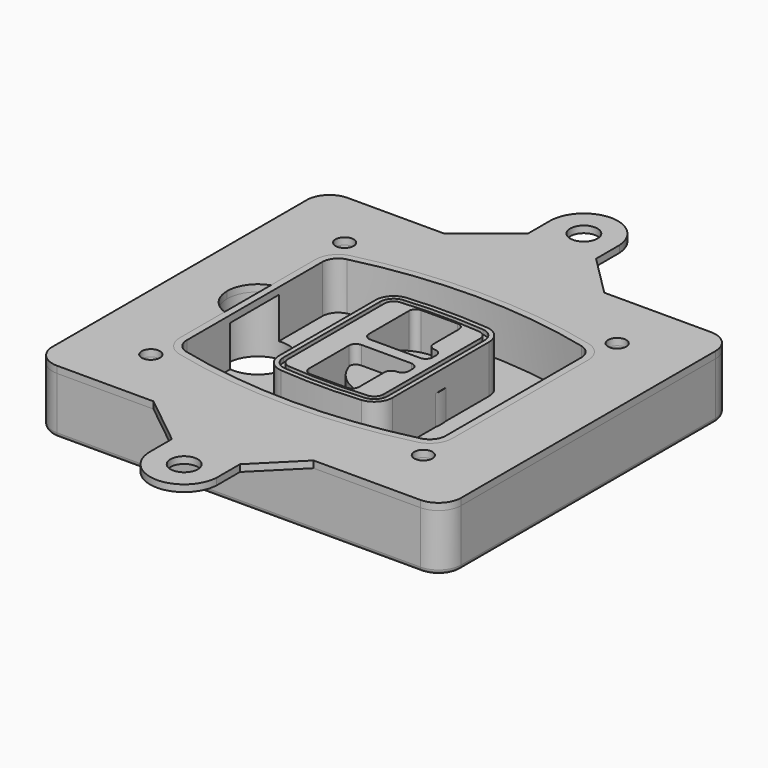
from build123d import *

# Parameters (mm, degrees)
F0_R      = 4
F1_DEPTH  = 25
F2_DEPTH  = 3
F3_DEPTH  = 18
F5_DEPTH  = 21
F6_DEPTH  = 2
F8_DEPTH  = 20
F9_DEPTH  = 16
F10_DEPTH = 25
F7_R      = 6
F7_R_2    = 4
F11_DEPTH = 6
F13_DEPTH = 9
F15_R     = 2
F16_R     = 6
F16_R_2   = 4
F17_DEPTH = 3


# Not quite as in the source:
# - a feature of the source that left no trace in its solid (it failed there, or was rolled back) is left out
# - a feature names something its author has since deleted; it is built from what else it names


with BuildPart() as f1:
    # F0 (on Top) → F1 (new body)
    with BuildSketch(Plane.XY):
        with BuildLine():
            ThreePointArc((-90, -70), (-87.0710678119, -77.0710678119), (-80, -80))
            Line((-80, -80), (80, -80))
            ThreePointArc((80, -80), (87.0710678119, -77.0710678119), (90, -70))
            Line((90, -70), (90, 70))
            ThreePointArc((90, 70), (87.0710678119, 77.0710678119), (80, 80))
            Line((80, 80), (-80, 80))
            ThreePointArc((-80, 80), (-87.0710678119, 77.0710678119), (-90, 70))
            Line((-90, 70), (-90, -70))
        make_face()
        with Locations((-60, -53.3333333333)):
            Circle(F0_R, mode=Mode.SUBTRACT)
        with Locations((60, -53.3333333333)):
            Circle(F0_R, mode=Mode.SUBTRACT)
        with Locations((-60, 53.3333333333)):
            Circle(F0_R, mode=Mode.SUBTRACT)
        with BuildLine():
            ThreePointArc((-64, 37.2990447398), (-61.0143011354, 45.9411029726), (-53.3306899286, 50.8970778549))
            ThreePointArc((-53.3306899286, 50.8970778549), (0, 57.3333333333), (53.3306899286, 50.8970778549))
            ThreePointArc((53.3306899286, 50.8970778549), (61.0143011354, 45.9411029726), (64, 37.2990447398))
            Line((64, 37.2990447398), (64, -37.2990447398))
            ThreePointArc((64, -37.2990447398), (61.0143011354, -45.9411029726), (53.3306899286, -50.8970778549))
            ThreePointArc((53.3306899286, -50.8970778549), (0, -57.3333333333), (-53.3306899286, -50.8970778549))
            ThreePointArc((-53.3306899286, -50.8970778549), (-61.0143011354, -45.9411029726), (-64, -37.2990447398))
            Line((-64, -37.2990447398), (-64, 37.2990447398))
        make_face(mode=Mode.SUBTRACT)
        with Locations((60, 53.3333333333)):
            Circle(F0_R, mode=Mode.SUBTRACT)
        with BuildLine():
            ThreePointArc((53.3306899286, 50.8970778549), (0, 57.3333333333), (-53.3306899286, 50.8970778549))
            ThreePointArc((-53.3306899286, 50.8970778549), (-61.0143011354, 45.9411029726), (-64, 37.2990447398))
            Line((-64, 37.2990447398), (-64, -37.2990447398))
            ThreePointArc((-64, -37.2990447398), (-61.0143011354, -45.9411029726), (-53.3306899286, -50.8970778549))
            ThreePointArc((-53.3306899286, -50.8970778549), (0, -57.3333333333), (53.3306899286, -50.8970778549))
            ThreePointArc((53.3306899286, -50.8970778549), (61.0143011354, -45.9411029726), (64, -37.2990447398))
            Line((64, -37.2990447398), (64, 37.2990447398))
            ThreePointArc((64, 37.2990447398), (61.0143011354, 45.9411029726), (53.3306899286, 50.8970778549))
        make_face()
        with BuildLine():
            Line((-60, -37.2990447398), (-60, 37.2990447398))
            ThreePointArc((-60, 37.2990447398), (-57.8673579538, 43.4719434775), (-52.3790642347, 47.0119255363))
            ThreePointArc((-52.3790642347, 47.0119255363), (0, 53.3333333333), (52.3790642347, 47.0119255363))
            ThreePointArc((52.3790642347, 47.0119255363), (57.8673579538, 43.4719434775), (60, 37.2990447398))
            Line((60, 37.2990447398), (60, -37.2990447398))
            ThreePointArc((60, -37.2990447398), (57.8673579538, -43.4719434775), (52.3790642347, -47.0119255363))
            ThreePointArc((52.3790642347, -47.0119255363), (0, -53.3333333333), (-52.3790642347, -47.0119255363))
            ThreePointArc((-52.3790642347, -47.0119255363), (-57.8673579538, -43.4719434775), (-60, -37.2990447398))
        make_face(mode=Mode.SUBTRACT)
        with BuildLine():
            ThreePointArc((-52.3790642347, 47.0119255363), (-57.8673579538, 43.4719434775), (-60, 37.2990447398))
            Line((-60, 37.2990447398), (-60, -37.2990447398))
            ThreePointArc((-60, -37.2990447398), (-57.8673579538, -43.4719434775), (-52.3790642347, -47.0119255363))
            ThreePointArc((-52.3790642347, -47.0119255363), (0, -53.3333333333), (52.3790642347, -47.0119255363))
            ThreePointArc((52.3790642347, -47.0119255363), (57.8673579538, -43.4719434775), (60, -37.2990447398))
            Line((60, -37.2990447398), (60, 37.2990447398))
            ThreePointArc((60, 37.2990447398), (57.8673579538, 43.4719434775), (52.3790642347, 47.0119255363))
            ThreePointArc((52.3790642347, 47.0119255363), (0, 53.3333333333), (-52.3790642347, 47.0119255363))
        make_face()
        with BuildLine():
            ThreePointArc((51.6653449643, 44.0980612973), (55.5071505677, 41.6200738562), (57, 37.2990447398))
            Line((57, 37.2990447398), (57, -37.2990447398))
            ThreePointArc((57, -37.2990447398), (55.5071505677, -41.6200738562), (51.6653449643, -44.0980612973))
            ThreePointArc((51.6653449643, -44.0980612973), (0, -50.3333333333), (-51.6653449643, -44.0980612973))
            ThreePointArc((-51.6653449643, -44.0980612973), (-55.5071505677, -41.6200738562), (-57, -37.2990447398))
            Line((-57, -37.2990447398), (-57, 37.2990447398))
            ThreePointArc((-57, 37.2990447398), (-55.5071505677, 41.6200738562), (-51.6653449643, 44.0980612973))
            ThreePointArc((-51.6653449643, 44.0980612973), (0, 50.3333333333), (51.6653449643, 44.0980612973))
        make_face(mode=Mode.SUBTRACT)
        with BuildLine():
            Line((57, -37.2990447398), (57, 37.2990447398))
            ThreePointArc((57, 37.2990447398), (55.5071505677, 41.6200738562), (51.6653449643, 44.0980612973))
            ThreePointArc((51.6653449643, 44.0980612973), (0, 50.3333333333), (-51.6653449643, 44.0980612973))
            ThreePointArc((-51.6653449643, 44.0980612973), (-55.5071505677, 41.6200738562), (-57, 37.2990447398))
            Line((-57, 37.2990447398), (-57, -37.2990447398))
            ThreePointArc((-57, -37.2990447398), (-55.5071505677, -41.6200738562), (-51.6653449643, -44.0980612973))
            ThreePointArc((-51.6653449643, -44.0980612973), (0, -50.3333333333), (51.6653449643, -44.0980612973))
            ThreePointArc((51.6653449643, -44.0980612973), (55.5071505677, -41.6200738562), (57, -37.2990447398))
        make_face()
    extrude(amount=-F1_DEPTH)

    # F0 (on Top) → F2 (join)
    with BuildSketch(Plane.XY):
        with BuildLine():
            ThreePointArc((-52.3790642347, 47.0119255363), (-57.8673579538, 43.4719434775), (-60, 37.2990447398))
            Line((-60, 37.2990447398), (-60, -37.2990447398))
            ThreePointArc((-60, -37.2990447398), (-57.8673579538, -43.4719434775), (-52.3790642347, -47.0119255363))
            ThreePointArc((-52.3790642347, -47.0119255363), (0, -53.3333333333), (52.3790642347, -47.0119255363))
            ThreePointArc((52.3790642347, -47.0119255363), (57.8673579538, -43.4719434775), (60, -37.2990447398))
            Line((60, -37.2990447398), (60, 37.2990447398))
            ThreePointArc((60, 37.2990447398), (57.8673579538, 43.4719434775), (52.3790642347, 47.0119255363))
            ThreePointArc((52.3790642347, 47.0119255363), (0, 53.3333333333), (-52.3790642347, 47.0119255363))
        make_face()
        with BuildLine():
            ThreePointArc((51.6653449643, 44.0980612973), (55.5071505677, 41.6200738562), (57, 37.2990447398))
            Line((57, 37.2990447398), (57, -37.2990447398))
            ThreePointArc((57, -37.2990447398), (55.5071505677, -41.6200738562), (51.6653449643, -44.0980612973))
            ThreePointArc((51.6653449643, -44.0980612973), (0, -50.3333333333), (-51.6653449643, -44.0980612973))
            ThreePointArc((-51.6653449643, -44.0980612973), (-55.5071505677, -41.6200738562), (-57, -37.2990447398))
            Line((-57, -37.2990447398), (-57, 37.2990447398))
            ThreePointArc((-57, 37.2990447398), (-55.5071505677, 41.6200738562), (-51.6653449643, 44.0980612973))
            ThreePointArc((-51.6653449643, 44.0980612973), (0, 50.3333333333), (51.6653449643, 44.0980612973))
        make_face(mode=Mode.SUBTRACT)
    extrude(amount=F2_DEPTH)

    # F0 (on Top) → F3 (cut)
    with BuildSketch(Plane.XY):
        with BuildLine():
            Line((57, -37.2990447398), (57, 37.2990447398))
            ThreePointArc((57, 37.2990447398), (55.5071505677, 41.6200738562), (51.6653449643, 44.0980612973))
            ThreePointArc((51.6653449643, 44.0980612973), (0, 50.3333333333), (-51.6653449643, 44.0980612973))
            ThreePointArc((-51.6653449643, 44.0980612973), (-55.5071505677, 41.6200738562), (-57, 37.2990447398))
            Line((-57, 37.2990447398), (-57, -37.2990447398))
            ThreePointArc((-57, -37.2990447398), (-55.5071505677, -41.6200738562), (-51.6653449643, -44.0980612973))
            ThreePointArc((-51.6653449643, -44.0980612973), (0, -50.3333333333), (51.6653449643, -44.0980612973))
            ThreePointArc((51.6653449643, -44.0980612973), (55.5071505677, -41.6200738562), (57, -37.2990447398))
        make_face()
    extrude(amount=-F3_DEPTH, mode=Mode.SUBTRACT)

    # F4 (on face) → F5 (join, through all)
    with BuildSketch(Plane.XY.offset(3)):
        with BuildLine():
            ThreePointArc((-25, -26.587695628), (-22.8992979869, -31.9912392117), (-17.7004291845, -34.5569740744))
            ThreePointArc((-17.7004291845, -34.5569740744), (0, -35.3333333333), (17.7004291845, -34.5569740744))
            ThreePointArc((17.7004291845, -34.5569740744), (22.8992979869, -31.9912392117), (25, -26.587695628))
            Line((25, -26.587695628), (25, 26.587695628))
            ThreePointArc((25, 26.587695628), (22.8992979869, 31.9912392117), (17.7004291845, 34.5569740744))
            ThreePointArc((17.7004291845, 34.5569740744), (0, 35.3333333333), (-17.7004291845, 34.5569740744))
            ThreePointArc((-17.7004291845, 34.5569740744), (-22.8992979869, 31.9912392117), (-25, 26.587695628))
            Line((-25, 26.587695628), (-25, -26.587695628))
        make_face()
        with BuildLine():
            ThreePointArc((17.5253218884, 32.5646544628), (21.4244734902, 30.6403533158), (23, 26.587695628))
            Line((23, 26.587695628), (23, -26.587695628))
            ThreePointArc((23, -26.587695628), (21.4244734902, -30.6403533158), (17.5253218884, -32.5646544628))
            ThreePointArc((17.5253218884, -32.5646544628), (0, -33.3333333333), (-17.5253218884, -32.5646544628))
            ThreePointArc((-17.5253218884, -32.5646544628), (-21.4244734902, -30.6403533158), (-23, -26.587695628))
            Line((-23, -26.587695628), (-23, 26.587695628))
            ThreePointArc((-23, 26.587695628), (-21.4244734902, 30.6403533158), (-17.5253218884, 32.5646544628))
            ThreePointArc((-17.5253218884, 32.5646544628), (0, 33.3333333333), (17.5253218884, 32.5646544628))
        make_face(mode=Mode.SUBTRACT)
        with BuildLine():
            Line((23, -26.587695628), (23, 26.587695628))
            ThreePointArc((23, 26.587695628), (21.4244734902, 30.6403533158), (17.5253218884, 32.5646544628))
            ThreePointArc((17.5253218884, 32.5646544628), (0, 33.3333333333), (-17.5253218884, 32.5646544628))
            ThreePointArc((-17.5253218884, 32.5646544628), (-21.4244734902, 30.6403533158), (-23, 26.587695628))
            Line((-23, 26.587695628), (-23, -26.587695628))
            ThreePointArc((-23, -26.587695628), (-21.4244734902, -30.6403533158), (-17.5253218884, -32.5646544628))
            ThreePointArc((-17.5253218884, -32.5646544628), (0, -33.3333333333), (17.5253218884, -32.5646544628))
            ThreePointArc((17.5253218884, -32.5646544628), (21.4244734902, -30.6403533158), (23, -26.587695628))
        make_face()
        with BuildLine():
            ThreePointArc((17.3502145923, 30.5723348512), (19.9496489934, 29.2894674198), (21, 26.587695628))
            Line((21, 26.587695628), (21, -26.587695628))
            ThreePointArc((21, -26.587695628), (19.9496489934, -29.2894674198), (17.3502145923, -30.5723348512))
            ThreePointArc((17.3502145923, -30.5723348512), (0, -31.3333333333), (-17.3502145923, -30.5723348512))
            ThreePointArc((-17.3502145923, -30.5723348512), (-19.9496489934, -29.2894674198), (-21, -26.587695628))
            Line((-21, -26.587695628), (-21, 26.587695628))
            ThreePointArc((-21, 26.587695628), (-19.9496489934, 29.2894674198), (-17.3502145923, 30.5723348512))
            ThreePointArc((-17.3502145923, 30.5723348512), (0, 31.3333333333), (17.3502145923, 30.5723348512))
        make_face(mode=Mode.SUBTRACT)
        with BuildLine():
            Line((21, -26.587695628), (21, 26.587695628))
            ThreePointArc((21, 26.587695628), (19.9496489934, 29.2894674198), (17.3502145923, 30.5723348512))
            ThreePointArc((17.3502145923, 30.5723348512), (0, 31.3333333333), (-17.3502145923, 30.5723348512))
            ThreePointArc((-17.3502145923, 30.5723348512), (-19.9496489934, 29.2894674198), (-21, 26.587695628))
            Line((-21, 26.587695628), (-21, -26.587695628))
            ThreePointArc((-21, -26.587695628), (-19.9496489934, -29.2894674198), (-17.3502145923, -30.5723348512))
            ThreePointArc((-17.3502145923, -30.5723348512), (0, -31.3333333333), (17.3502145923, -30.5723348512))
            ThreePointArc((17.3502145923, -30.5723348512), (19.9496489934, -29.2894674198), (21, -26.587695628))
        make_face()
        with BuildLine():
            Line((-8, -2.5), (14, -2.5))
            ThreePointArc((14, -2.5), (16.1213203436, -3.3786796564), (17, -5.5))
            Line((17, -5.5), (17, -7.5))
            ThreePointArc((17, -7.5), (16.1213203436, -9.6213203436), (14, -10.5))
            ThreePointArc((14, -10.5), (11.8786796564, -11.3786796564), (11, -13.5))
            Line((11, -13.5), (11, -27.5))
            ThreePointArc((11, -27.5), (10.1213203436, -29.6213203436), (8, -30.5))
            Line((8, -30.5), (-8, -30.5))
            ThreePointArc((-8, -30.5), (-10.1213203436, -29.6213203436), (-11, -27.5))
            Line((-11, -27.5), (-11, -5.5))
            ThreePointArc((-11, -5.5), (-10.1213203436, -3.3786796564), (-8, -2.5))
        make_face(mode=Mode.SUBTRACT)
        with BuildLine():
            ThreePointArc((-8, 2.5), (-10.1213203436, 3.3786796564), (-11, 5.5))
            Line((-11, 5.5), (-11, 27.5))
            ThreePointArc((-11, 27.5), (-10.1213203436, 29.6213203436), (-8, 30.5))
            Line((-8, 30.5), (8, 30.5))
            ThreePointArc((8, 30.5), (10.1213203436, 29.6213203436), (11, 27.5))
            Line((11, 27.5), (11, 13.5))
            ThreePointArc((11, 13.5), (11.8786796564, 11.3786796564), (14, 10.5))
            ThreePointArc((14, 10.5), (16.1213203436, 9.6213203436), (17, 7.5))
            Line((17, 7.5), (17, 5.5))
            ThreePointArc((17, 5.5), (16.1213203436, 3.3786796564), (14, 2.5))
            Line((14, 2.5), (-8, 2.5))
        make_face(mode=Mode.SUBTRACT)
    extrude(amount=-F5_DEPTH)

    # F4 (on face) → F6 (cut)
    with BuildSketch(Plane.XY.offset(3)):
        with BuildLine():
            Line((23, -26.587695628), (23, 26.587695628))
            ThreePointArc((23, 26.587695628), (21.4244734902, 30.6403533158), (17.5253218884, 32.5646544628))
            ThreePointArc((17.5253218884, 32.5646544628), (0, 33.3333333333), (-17.5253218884, 32.5646544628))
            ThreePointArc((-17.5253218884, 32.5646544628), (-21.4244734902, 30.6403533158), (-23, 26.587695628))
            Line((-23, 26.587695628), (-23, -26.587695628))
            ThreePointArc((-23, -26.587695628), (-21.4244734902, -30.6403533158), (-17.5253218884, -32.5646544628))
            ThreePointArc((-17.5253218884, -32.5646544628), (0, -33.3333333333), (17.5253218884, -32.5646544628))
            ThreePointArc((17.5253218884, -32.5646544628), (21.4244734902, -30.6403533158), (23, -26.587695628))
        make_face()
        with BuildLine():
            ThreePointArc((17.3502145923, 30.5723348512), (19.9496489934, 29.2894674198), (21, 26.587695628))
            Line((21, 26.587695628), (21, -26.587695628))
            ThreePointArc((21, -26.587695628), (19.9496489934, -29.2894674198), (17.3502145923, -30.5723348512))
            ThreePointArc((17.3502145923, -30.5723348512), (0, -31.3333333333), (-17.3502145923, -30.5723348512))
            ThreePointArc((-17.3502145923, -30.5723348512), (-19.9496489934, -29.2894674198), (-21, -26.587695628))
            Line((-21, -26.587695628), (-21, 26.587695628))
            ThreePointArc((-21, 26.587695628), (-19.9496489934, 29.2894674198), (-17.3502145923, 30.5723348512))
            ThreePointArc((-17.3502145923, 30.5723348512), (0, 31.3333333333), (17.3502145923, 30.5723348512))
        make_face(mode=Mode.SUBTRACT)
    extrude(amount=-F6_DEPTH, mode=Mode.SUBTRACT)

    # F7 (on face) → F8 (join)
    with BuildSketch(Plane(origin=(0, 0, -25), x_dir=(1, 0, 0), z_dir=(0, 0, -1))):
        with BuildLine():
            ThreePointArc((-6.71157564, 0), (6.7567035675, 13.4682792075), (20.224982775, 0))
            Line((20.224982775, 0), (25.224982775, 0))
            ThreePointArc((25.224982775, 0), (6.7567035675, 18.4682792075), (-11.71157564, 0))
            Line((-11.71157564, 0), (-6.71157564, 0))
        make_face()
        with BuildLine():
            Line((-6.71157564, 0), (20.224982775, 0))
            ThreePointArc((20.224982775, 0), (6.7567035675, 13.4682792075), (-6.71157564, 0))
        make_face()
        with BuildLine():
            ThreePointArc((-6.71157564, 0), (6.7567035675, -13.4682792075), (20.224982775, 0))
            Line((20.224982775, 0), (-6.71157564, 0))
        make_face()
        with BuildLine():
            Line((25.224982775, 0), (20.224982775, 0))
            ThreePointArc((20.224982775, 0), (6.7567035675, -13.4682792075), (-6.71157564, 0))
            Line((-6.71157564, 0), (-11.71157564, 0))
            ThreePointArc((-11.71157564, 0), (6.7567035675, -18.4682792075), (25.224982775, 0))
        make_face()
    extrude(amount=-F8_DEPTH)

    # F7 (on face) → F9 (cut)
    with BuildSketch(Plane(origin=(0, 0, -25), x_dir=(1, 0, 0), z_dir=(0, 0, -1))):
        with BuildLine():
            Line((-6.71157564, 0), (20.224982775, 0))
            ThreePointArc((20.224982775, 0), (6.7567035675, 13.4682792075), (-6.71157564, 0))
        make_face()
        with BuildLine():
            ThreePointArc((-6.71157564, 0), (6.7567035675, -13.4682792075), (20.224982775, 0))
            Line((20.224982775, 0), (-6.71157564, 0))
        make_face()
    extrude(amount=-F9_DEPTH, mode=Mode.SUBTRACT)

    # F7 (on face) → F10 (cut)
    with BuildSketch(Plane(origin=(0, 0, -25), x_dir=(1, 0, 0), z_dir=(0, 0, -1))):
        with BuildLine():
            Line((-69.0318229325, 0), (-42.0952645175, 0))
            ThreePointArc((-42.0952645175, 0), (-55.563543725, 13.4682792075), (-69.0318229325, 0))
        make_face()
        with BuildLine():
            ThreePointArc((-69.0318229325, 0), (-55.563543725, -13.4682792075), (-42.0952645175, 0))
            Line((-42.0952645175, 0), (-69.0318229325, 0))
        make_face()
    extrude(amount=-F10_DEPTH, mode=Mode.SUBTRACT)

    # F7 (on face) → F11 (cut)
    with BuildSketch(Plane(origin=(0, 0, -25), x_dir=(1, 0, 0), z_dir=(0, 0, -1))):
        with Locations((60, -53.3333333333)):
            Circle(F7_R)
        with Locations((60, -53.3333333333)):
            Circle(F7_R_2, mode=Mode.SUBTRACT)
        with Locations((-60, -53.3333333333)):
            Circle(F7_R)
        with Locations((-60, -53.3333333333)):
            Circle(F7_R_2, mode=Mode.SUBTRACT)
        with Locations((-60, 53.3333333333)):
            Circle(F7_R)
        with Locations((-60, 53.3333333333)):
            Circle(F7_R_2, mode=Mode.SUBTRACT)
        with Locations((60, 53.3333333333)):
            Circle(F7_R)
        with Locations((60, 53.3333333333)):
            Circle(F7_R_2, mode=Mode.SUBTRACT)
    extrude(amount=-F11_DEPTH, mode=Mode.SUBTRACT)

    # F12 (on face) → F13 (cut, through all)
    with BuildSketch(Plane(origin=(0, 0, -9), x_dir=(1, 0, 0), z_dir=(0, 0, -1))):
        with BuildLine():
            ThreePointArc((20.224982775, 0), (20.1663399806, 1.2554664788), (19.9909222755, 2.5))
            Line((19.9909222755, 2.5), (14, 2.5))
            ThreePointArc((14, 2.5), (16.1213203436, 3.3786796564), (17, 5.5))
            Line((17, 5.5), (17, 7.5))
            ThreePointArc((17, 7.5), (16.1213203436, 9.6213203436), (14, 10.5))
            ThreePointArc((14, 10.5), (12.1627255951, 11.1284134507), (11.0951631559, 12.750384826))
            ThreePointArc((11.0951631559, 12.750384826), (11.0476113807, 12.7664660322), (11, 12.7823698976))
            Line((11, 12.7823698976), (11, -12.7823698976))
            ThreePointArc((11, -12.7823698976), (11.0476113807, -12.7664660322), (11.0951631559, -12.750384826))
            ThreePointArc((11.0951631559, -12.750384826), (12.1627255951, -11.1284134507), (14, -10.5))
            ThreePointArc((14, -10.5), (16.1213203436, -9.6213203436), (17, -7.5))
            Line((17, -7.5), (17, -5.5))
            ThreePointArc((17, -5.5), (16.1213203436, -3.3786796564), (14, -2.5))
            Line((14, -2.5), (19.9909222755, -2.5))
            ThreePointArc((19.9909222755, -2.5), (20.1663399806, -1.2554664788), (20.224982775, 0))
        make_face()
    extrude(amount=F13_DEPTH, mode=Mode.SUBTRACT)

    # F15
    f15_edges = [f1.edges().sort_by_distance(p)[0] for p in [
        (0, -80, -25),
        (-87.071068, -77.071068, -25),
        (-90, 0, -25),
        (-87.071068, 77.071068, -25),
        (87.071068, -77.071068, -25),
        (0, 80, -25),
        (90, 0, -25),
        (87.071068, 77.071068, -25),
    ]]
    fillet(f15_edges, radius=F15_R)


with BuildPart() as f17:
    # F16 (on face) → F17 (new body, through all)
    with BuildSketch(Plane.XY):
        with BuildLine():
            Line((-15, 98), (-37.4856255949, 80))
            Line((-37.4856255949, 80), (32.974961694, 80))
            Line((32.974961694, 80), (14.974961694, 98))
            Line((14.974961694, 98), (14.974961694, 110.8663268794))
            ThreePointArc((14.974961694, 110.8663268794), (-0.4333443142, 124.9937391169), (-15, 110))
            Line((-15, 110), (-15, 98))
        make_face()
        with Locations((0, 110)):
            Circle(F16_R, mode=Mode.SUBTRACT)
        with BuildLine():
            Line((32.974961694, -80), (-37.4856255949, -80))
            Line((-37.4856255949, -80), (-15, -98))
            Line((-15, -98), (-15, -110))
            ThreePointArc((-15, -110), (-0.4333443142, -124.9937391169), (14.974961694, -110.8663268794))
            Line((14.974961694, -110.8663268794), (14.974961694, -98))
            Line((14.974961694, -98), (32.974961694, -80))
        make_face()
        with Locations((0, -110)):
            Circle(F16_R, mode=Mode.SUBTRACT)
        with BuildLine():
            Line((32.974961694, 80), (-37.4856255949, 80))
            Line((-37.4856255949, 80), (-80, 80))
            ThreePointArc((-80, 80), (-87.0710678119, 77.0710678119), (-90, 70))
            Line((-90, 70), (-90, -70))
            ThreePointArc((-90, -70), (-87.0710678119, -77.0710678119), (-80, -80))
            Line((-80, -80), (-37.4856255949, -80))
            Line((-37.4856255949, -80), (32.974961694, -80))
            Line((32.974961694, -80), (80, -80))
            ThreePointArc((80, -80), (87.0710678119, -77.0710678119), (90, -70))
            Line((90, -70), (90, 70))
            ThreePointArc((90, 70), (87.0710678119, 77.0710678119), (80, 80))
            Line((80, 80), (32.974961694, 80))
        make_face()
        with Locations((-60, -53.3333333333)):
            Circle(F16_R_2, mode=Mode.SUBTRACT)
        with BuildLine():
            ThreePointArc((-60, 37.2990447398), (-57.8673579538, 43.4719434775), (-52.3790642347, 47.0119255363))
            ThreePointArc((-52.3790642347, 47.0119255363), (0, 53.3333333333), (52.3790642347, 47.0119255363))
            ThreePointArc((52.3790642347, 47.0119255363), (57.8673579538, 43.4719434775), (60, 37.2990447398))
            Line((60, 37.2990447398), (60, -37.2990447398))
            ThreePointArc((60, -37.2990447398), (57.8673579538, -43.4719434775), (52.3790642347, -47.0119255363))
            ThreePointArc((52.3790642347, -47.0119255363), (0, -53.3333333333), (-52.3790642347, -47.0119255363))
            ThreePointArc((-52.3790642347, -47.0119255363), (-57.8673579538, -43.4719434775), (-60, -37.2990447398))
            Line((-60, -37.2990447398), (-60, -12.7166190685))
            ThreePointArc((-60, -12.7166190685), (-66.5441169481, -7.798817635), (-69.0318229325, 0))
            ThreePointArc((-69.0318229325, 0), (-66.5441169481, 7.798817635), (-60, 12.7166190685))
            Line((-60, 12.7166190685), (-60, 37.2990447398))
        make_face(mode=Mode.SUBTRACT)
        with Locations((60, -53.3333333333)):
            Circle(F16_R_2, mode=Mode.SUBTRACT)
        with Locations((-60, 53.3333333333)):
            Circle(F16_R_2, mode=Mode.SUBTRACT)
        with Locations((60, 53.3333333333)):
            Circle(F16_R_2, mode=Mode.SUBTRACT)
    extrude(amount=F17_DEPTH)


solid = Compound([f1.part, f17.part])
